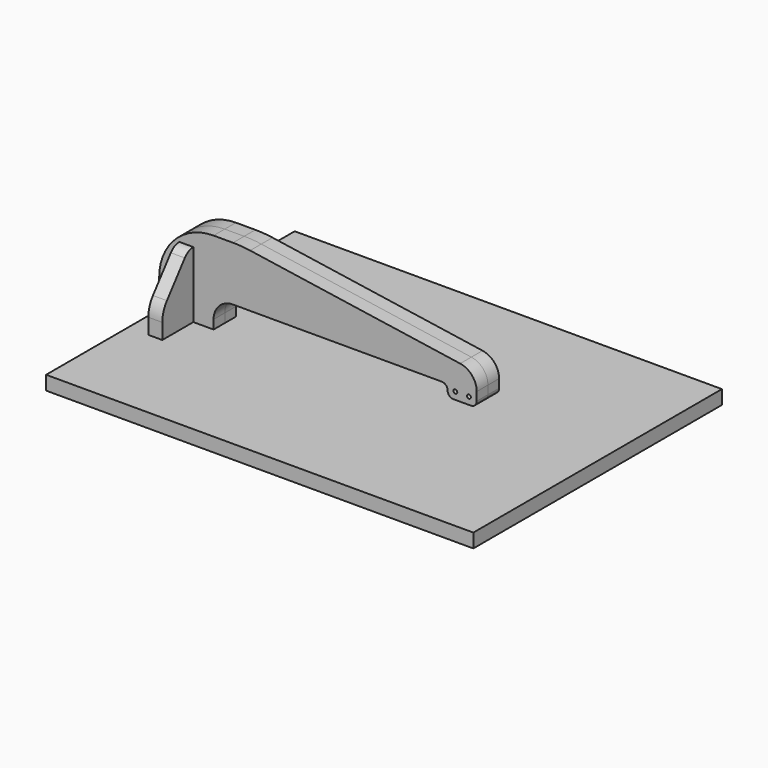
from build123d import *

# Parameters (mm, degrees)
F0_R     = 2.5
F1_DEPTH = 18
F3_W     = 550
F3_H     = 400
F4_DEPTH = 18
F6_START = -26
F6_DEPTH = 18


with BuildPart() as f1:
    # F0 (on Front) → F1 (new body)
    with BuildSketch(Plane.XZ):
        with BuildLine():
            Line((0, 36.5), (0, 0))
            Line((0, 0), (70, 0))
            Line((70, 0), (70, 11.5))
            ThreePointArc((70, 11.5), (77.3223304703, 29.1776695297), (95, 36.5))
            Line((95, 36.5), (363.75, 36.5))
            ThreePointArc((363.75, 36.5), (369.0533008589, 34.3033008589), (371.25, 29))
            ThreePointArc((371.25, 29), (373.4466991411, 23.6966991411), (378.75, 21.5))
            Line((378.75, 21.5), (401.25, 21.5))
            ThreePointArc((401.25, 21.5), (406.5533008589, 23.6966991411), (408.75, 29))
            Line((408.75, 29), (408.75, 39.9422265221))
            ThreePointArc((408.75, 39.9422265221), (402.6829832168, 56.26834506), (387.4266282789, 64.670396784))
            Line((387.4266282789, 64.670396784), (117.0597696734, 104.8690215711))
            ThreePointArc((117.0597696734, 104.8690215711), (106.0599901524, 106.0916996956), (95, 106.5))
            Line((95, 106.5), (70, 106.5))
            ThreePointArc((70, 106.5), (20.5025253169, 85.9974746831), (0, 36.5))
        make_face()
        with Locations((381.25, 31)):
            Circle(F0_R, mode=Mode.SUBTRACT)
        with Locations((398.75, 31)):
            Circle(F0_R, mode=Mode.SUBTRACT)
    extrude(amount=F1_DEPTH)


with BuildPart() as f2_1:
    # F2: copy of F1
    add(f1.part.moved(Location((0, 18, 0))))


with BuildPart() as f4:
    # F3 (on face) → F4 (new body)
    with BuildSketch(Plane(origin=(0, 0, 0), x_dir=(1, 0, 0), z_dir=(0, 0, -1))):
        with Locations((275, 0)):
            Rectangle(F3_W, F3_H)
    extrude(amount=F4_DEPTH)


with BuildPart() as f6:
    # F5 (on face) → F6 (new body)
    with BuildSketch(Plane(origin=(0, 0, 0), x_dir=(0, -1, 0), z_dir=(-1, 0, 0)).offset(F6_START)):
        with BuildLine():
            Line((-68, 0), (-18, 0))
            Line((-18, 0), (-18, 85))
            ThreePointArc((-18, 85), (-25.6586397747, 83.2351592557), (-31.7725618899, 78.2965984916))
            Line((-31.7725618899, 78.2965984916), (-60.5451237799, 41.5931969831))
            ThreePointArc((-60.5451237799, 41.5931969831), (-66.0838278642, 31.4219233867), (-68, 20))
            Line((-68, 20), (-68, 0))
        make_face()
    extrude(amount=-F6_DEPTH)


with BuildPart() as f6b:
    # F5 (on face) → F6, piece 2 (new body)
    with BuildSketch(Plane(origin=(0, 0, 0), x_dir=(0, -1, 0), z_dir=(-1, 0, 0)).offset(F6_START)):
        with BuildLine():
            Line((18, 85), (18, 0))
            Line((18, 0), (68, 0))
            Line((68, 0), (68, 20))
            ThreePointArc((68, 20), (66.0838278642, 31.4219233867), (60.5451237799, 41.5931969831))
            Line((60.5451237799, 41.5931969831), (31.7725618899, 78.2965984916))
            ThreePointArc((31.7725618899, 78.2965984916), (25.6586397747, 83.2351592557), (18, 85))
        make_face()
    extrude(amount=-F6_DEPTH)


solid = Compound([f1.part, f2_1.part, f4.part, f6.part, f6b.part])
